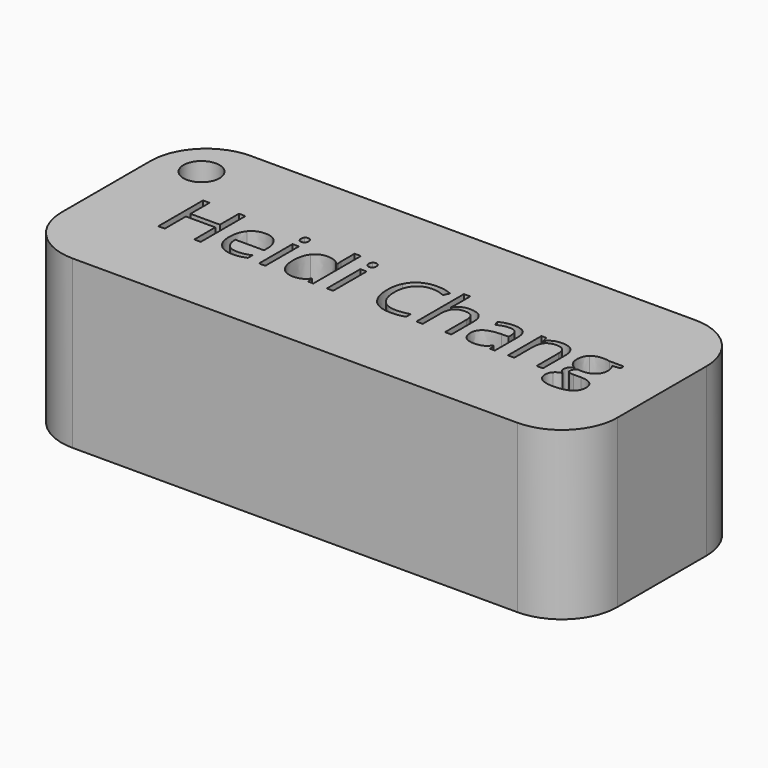
from build123d import *

# Parameters (mm, degrees)
F0_W     = 1.1420084165
F0_H     = 7.5363753885
F0_R     = 3.2310407431
F1_DEPTH = 30


with BuildPart() as f1:
    # F0 (on Top) → F1 (new body)
    with BuildSketch(Plane.XY):
        with BuildLine():
            Line((90, 41.9395349271), (10, 41.9395349271))
            ThreePointArc((10, 41.9395349271), (2.9289321881, 39.0106027389), (0, 31.9395349271))
            Line((0, 31.9395349271), (0, 11.9395349271))
            ThreePointArc((0, 11.9395349271), (2.9289321881, 4.8684671152), (10, 1.9395349271))
            Line((10, 1.9395349271), (90, 1.9395349271))
            ThreePointArc((90, 1.9395349271), (97.0710678119, 4.8684671152), (100, 11.9395349271))
            Line((100, 11.9395349271), (100, 31.9395349271))
            ThreePointArc((100, 31.9395349271), (97.0710678119, 39.0106027389), (90, 41.9395349271))
        make_face()
        with BuildLine():
            add(Edge.make_bspline(
                [(27.9621376159, 17.0902174011), (27.4230392305, 16.9757965193), (26.6594998845, 16.9757965193)],
                knots=[0, 0, 0, 1, 1, 1], degree=2))
            add(Edge.make_bspline(
                [(26.6594998845, 16.9757965193), (24.9893950904, 16.9757965193), (24.022318599, 17.9945824477)],
                knots=[0, 0, 0, 1, 1, 1], degree=2))
            add(Edge.make_bspline(
                [(24.022318599, 17.9945824477), (23.0552421075, 19.0133683762), (23.0552421075, 20.8198980678)],
                knots=[0, 0, 0, 1, 1, 1], degree=2))
            add(Edge.make_bspline(
                [(23.0552421075, 20.8198980678), (23.0552421075, 22.6440309721), (23.9530059494, 23.7167267391)],
                knots=[0, 0, 0, 1, 1, 1], degree=2))
            add(Edge.make_bspline(
                [(23.9530059494, 23.7167267391), (24.8507697913, 24.789422506), (26.3646460737, 24.789422506)],
                knots=[0, 0, 0, 1, 1, 1], degree=2))
            add(Edge.make_bspline(
                [(26.3646460737, 24.789422506), (27.7795042854, 24.789422506), (28.6046548753, 23.8575524397)],
                knots=[0, 0, 0, 1, 1, 1], degree=2))
            add(Edge.make_bspline(
                [(28.6046548753, 23.8575524397), (29.4298054653, 22.9256823735), (29.4298054653, 21.3986036816)],
                knots=[0, 0, 0, 1, 1, 1], degree=2))
            Line((29.4298054653, 21.3986036816), (29.4298054653, 20.6768719656))
            Line((29.4298054653, 20.6768719656), (24.2390581539, 20.6768719656))
            add(Edge.make_bspline(
                [(24.2390581539, 20.6768719656), (24.2742645791, 19.3500298169), (24.9101806338, 18.6624043252)],
                knots=[0, 0, 0, 1, 1, 1], degree=2))
            add(Edge.make_bspline(
                [(24.9101806338, 18.6624043252), (25.5460966885, 17.9747788336), (26.7013075144, 17.9747788336)],
                knots=[0, 0, 0, 1, 1, 1], degree=2))
            add(Edge.make_bspline(
                [(26.7013075144, 17.9747788336), (27.9181295845, 17.9747788336), (29.106346434, 18.483071597)],
                knots=[0, 0, 0, 1, 1, 1], degree=2))
            Line((29.106346434, 18.483071597), (29.106346434, 17.4642856686))
            add(Edge.make_bspline(
                [(29.106346434, 17.4642856686), (28.5012360014, 17.2046382829), (27.9621376159, 17.0902174011)],
                knots=[0, 0, 0, 1, 1, 1], degree=2))
        make_face(mode=Mode.SUBTRACT)
        with Locations((31.9481650659, 20.8826095127)):
            Rectangle(F0_W, F0_H, mode=Mode.SUBTRACT)
        with Locations((44.1405901835, 20.8826095127)):
            Rectangle(F0_W, F0_H, mode=Mode.SUBTRACT)
        with BuildLine():
            Line((73.8009031907, 17.1144218184), (72.9537485849, 17.1144218184))
            Line((72.9537485849, 17.1144218184), (72.7271072229, 18.1882177862))
            Line((72.7271072229, 18.1882177862), (72.6720971836, 18.1882177862))
            add(Edge.make_bspline(
                [(72.6720971836, 18.1882177862), (72.1087943808, 17.4796884796), (71.5487921804, 17.2277424994)],
                knots=[0, 0, 0, 1, 1, 1], degree=2))
            add(Edge.make_bspline(
                [(71.5487921804, 17.2277424994), (70.98878998, 16.9757965193), (70.148236579, 16.9757965193)],
                knots=[0, 0, 0, 1, 1, 1], degree=2))
            add(Edge.make_bspline(
                [(70.148236579, 16.9757965193), (69.0282321782, 16.9757965193), (68.3923161235, 17.5545021331)],
                knots=[0, 0, 0, 1, 1, 1], degree=2))
            add(Edge.make_bspline(
                [(68.3923161235, 17.5545021331), (67.7564000688, 18.1332077468), (67.7564000688, 19.1982021083)],
                knots=[0, 0, 0, 1, 1, 1], degree=2))
            add(Edge.make_bspline(
                [(67.7564000688, 19.1982021083), (67.7564000688, 21.4800185398), (71.4068662789, 21.5900386185)],
                knots=[0, 0, 0, 1, 1, 1], degree=2))
            Line((71.4068662789, 21.5900386185), (72.685299593, 21.6318462484))
            Line((72.685299593, 21.6318462484), (72.685299593, 22.1005317835))
            add(Edge.make_bspline(
                [(72.685299593, 22.1005317835), (72.685299593, 22.9872936175), (72.3046301208, 23.4097707196)],
                knots=[0, 0, 0, 1, 1, 1], degree=2))
            add(Edge.make_bspline(
                [(72.3046301208, 23.4097707196), (71.9239606486, 23.8322478217), (71.0834072476, 23.8322478217)],
                knots=[0, 0, 0, 1, 1, 1], degree=2))
            add(Edge.make_bspline(
                [(71.0834072476, 23.8322478217), (70.1416353743, 23.8322478217), (68.9534185247, 23.2557426094)],
                knots=[0, 0, 0, 1, 1, 1], degree=2))
            Line((68.9534185247, 23.2557426094), (68.601354273, 24.129302034))
            add(Edge.make_bspline(
                [(68.601354273, 24.129302034), (69.158055871, 24.4307570496), (69.8214769454, 24.6023883723)],
                knots=[0, 0, 0, 1, 1, 1], degree=2))
            add(Edge.make_bspline(
                [(69.8214769454, 24.6023883723), (70.4848980197, 24.774019695), (71.153820098, 24.774019695)],
                knots=[0, 0, 0, 1, 1, 1], degree=2))
            add(Edge.make_bspline(
                [(71.153820098, 24.774019695), (72.5004658608, 24.774019695), (73.1506845257, 24.1766106679)],
                knots=[0, 0, 0, 1, 1, 1], degree=2))
            add(Edge.make_bspline(
                [(73.1506845257, 24.1766106679), (73.8009031907, 23.5792016407), (73.8009031907, 22.2589606968)],
                knots=[0, 0, 0, 1, 1, 1], degree=2))
            Line((73.8009031907, 22.2589606968), (73.8009031907, 17.1144218184))
        make_face(mode=Mode.SUBTRACT)
        with BuildLine():
            Line((88.3565595979, 24.6507972069), (90.9618350607, 24.6507972069))
            Line((90.9618350607, 24.6507972069), (90.9618350607, 23.9290654909))
            Line((90.9618350607, 23.9290654909), (89.5667804633, 23.7640353729))
            add(Edge.make_bspline(
                [(89.5667804633, 23.7640353729), (89.7582154001, 23.5241916014), (89.9100431087, 23.1347205229)],
                knots=[0, 0, 0, 1, 1, 1], degree=2))
            add(Edge.make_bspline(
                [(89.9100431087, 23.1347205229), (90.0618708172, 22.7452494444), (90.0618708172, 22.2589606968)],
                knots=[0, 0, 0, 1, 1, 1], degree=2))
            add(Edge.make_bspline(
                [(90.0618708172, 22.2589606968), (90.0618708172, 21.1499583038), (89.304932676, 20.4898378318)],
                knots=[0, 0, 0, 1, 1, 1], degree=2))
            add(Edge.make_bspline(
                [(89.304932676, 20.4898378318), (88.5479945348, 19.8297173598), (87.2277535909, 19.8297173598)],
                knots=[0, 0, 0, 1, 1, 1], degree=2))
            add(Edge.make_bspline(
                [(87.2277535909, 19.8297173598), (86.8910921501, 19.8297173598), (86.5962383393, 19.8847273992)],
                knots=[0, 0, 0, 1, 1, 1], degree=2))
            add(Edge.make_bspline(
                [(86.5962383393, 19.8847273992), (85.8679054186, 19.4996571238), (85.8679054186, 18.9165507069)],
                knots=[0, 0, 0, 1, 1, 1], degree=2))
            add(Edge.make_bspline(
                [(85.8679054186, 18.9165507069), (85.8679054186, 18.6062940851), (86.1220518003, 18.4588671797)],
                knots=[0, 0, 0, 1, 1, 1], degree=2))
            add(Edge.make_bspline(
                [(86.1220518003, 18.4588671797), (86.376198182, 18.3114402743), (86.9945110241, 18.3114402743)],
                knots=[0, 0, 0, 1, 1, 1], degree=2))
            Line((86.9945110241, 18.3114402743), (88.3279543775, 18.3114402743))
            add(Edge.make_bspline(
                [(88.3279543775, 18.3114402743), (89.5535780538, 18.3114402743), (90.2092977227, 17.7954461053)],
                knots=[0, 0, 0, 1, 1, 1], degree=2))
            add(Edge.make_bspline(
                [(90.2092977227, 17.7954461053), (90.8650173915, 17.2794519364), (90.8650173915, 16.2958724331)],
                knots=[0, 0, 0, 1, 1, 1], degree=2))
            add(Edge.make_bspline(
                [(90.8650173915, 16.2958724331), (90.8650173915, 15.0438439379), (89.8616342741, 14.3870240683)],
                knots=[0, 0, 0, 1, 1, 1], degree=2))
            add(Edge.make_bspline(
                [(89.8616342741, 14.3870240683), (88.8582511567, 13.7302041987), (86.93289978, 13.7302041987)],
                knots=[0, 0, 0, 1, 1, 1], degree=2))
            add(Edge.make_bspline(
                [(86.93289978, 13.7302041987), (85.4542299228, 13.7302041987), (84.6532837501, 14.280304592)],
                knots=[0, 0, 0, 1, 1, 1], degree=2))
            add(Edge.make_bspline(
                [(84.6532837501, 14.280304592), (83.8523375774, 14.8304049853), (83.8523375774, 15.8359885043)],
                knots=[0, 0, 0, 1, 1, 1], degree=2))
            add(Edge.make_bspline(
                [(83.8523375774, 15.8359885043), (83.8523375774, 16.5225137952), (84.2924178921, 17.0253055547)],
                knots=[0, 0, 0, 1, 1, 1], degree=2))
            add(Edge.make_bspline(
                [(84.2924178921, 17.0253055547), (84.7324982067, 17.5280973142), (85.5290435763, 17.7063298416)],
                knots=[0, 0, 0, 1, 1, 1], degree=2))
            add(Edge.make_bspline(
                [(85.5290435763, 17.7063298416), (85.2407909702, 17.8361535344), (85.0449552302, 18.1112037311)],
                knots=[0, 0, 0, 1, 1, 1], degree=2))
            add(Edge.make_bspline(
                [(85.0449552302, 18.1112037311), (84.8491194901, 18.3862539278), (84.8491194901, 18.7515205889)],
                knots=[0, 0, 0, 1, 1, 1], degree=2))
            add(Edge.make_bspline(
                [(84.8491194901, 18.7515205889), (84.8491194901, 19.1629956831), (85.0691596475, 19.473252305)],
                knots=[0, 0, 0, 1, 1, 1], degree=2))
            add(Edge.make_bspline(
                [(85.0691596475, 19.473252305), (85.2891998048, 19.7835089268), (85.7644865446, 20.0717615329)],
                knots=[0, 0, 0, 1, 1, 1], degree=2))
            add(Edge.make_bspline(
                [(85.7644865446, 20.0717615329), (85.1791797261, 20.3116053044), (84.8117126634, 20.8892107174)],
                knots=[0, 0, 0, 1, 1, 1], degree=2))
            add(Edge.make_bspline(
                [(84.8117126634, 20.8892107174), (84.4442456006, 21.4668161304), (84.4442456006, 22.2105518621)],
                knots=[0, 0, 0, 1, 1, 1], degree=2))
            add(Edge.make_bspline(
                [(84.4442456006, 22.2105518621), (84.4442456006, 23.4471775463), (85.1868811316, 24.1183000262)],
                knots=[0, 0, 0, 1, 1, 1], degree=2))
            add(Edge.make_bspline(
                [(85.1868811316, 24.1183000262), (85.9295166626, 24.789422506), (87.2893648349, 24.789422506)],
                knots=[0, 0, 0, 1, 1, 1], degree=2))
            add(Edge.make_bspline(
                [(87.2893648349, 24.789422506), (87.8812728581, 24.789422506), (88.3565595979, 24.6507972069)],
                knots=[0, 0, 0, 1, 1, 1], degree=2))
        make_face(mode=Mode.SUBTRACT)
        with BuildLine():
            Line((82.4506817752, 17.1144218184), (81.3086733587, 17.1144218184))
            Line((81.3086733587, 17.1144218184), (81.3086733587, 21.9905117048))
            add(Edge.make_bspline(
                [(81.3086733587, 21.9905117048), (81.3086733587, 22.9102795624), (80.889496859, 23.3646624873)],
                knots=[0, 0, 0, 1, 1, 1], degree=2))
            add(Edge.make_bspline(
                [(80.889496859, 23.3646624873), (80.4703203593, 23.8190454122), (79.574756919, 23.8190454122)],
                knots=[0, 0, 0, 1, 1, 1], degree=2))
            add(Edge.make_bspline(
                [(79.574756919, 23.8190454122), (78.3931412741, 23.8190454122), (77.8430408808, 23.1798287552)],
                knots=[0, 0, 0, 1, 1, 1], degree=2))
            add(Edge.make_bspline(
                [(77.8430408808, 23.1798287552), (77.2929404875, 22.5406120981), (77.2929404875, 21.0685434456)],
                knots=[0, 0, 0, 1, 1, 1], degree=2))
            Line((77.2929404875, 21.0685434456), (77.2929404875, 17.1144218184))
            Line((77.2929404875, 17.1144218184), (76.1509320709, 17.1144218184))
            Line((76.1509320709, 17.1144218184), (76.1509320709, 24.6507972069))
            Line((76.1509320709, 24.6507972069), (77.0795015349, 24.6507972069))
            Line((77.0795015349, 24.6507972069), (77.264335267, 23.618808869))
            Line((77.264335267, 23.618808869), (77.3193453063, 23.618808869))
            add(Edge.make_bspline(
                [(77.3193453063, 23.618808869), (77.6714095581, 24.1755104671), (78.3040250104, 24.4824664866)],
                knots=[0, 0, 0, 1, 1, 1], degree=2))
            add(Edge.make_bspline(
                [(78.3040250104, 24.4824664866), (78.9366404627, 24.789422506), (79.7133822181, 24.789422506)],
                knots=[0, 0, 0, 1, 1, 1], degree=2))
            add(Edge.make_bspline(
                [(79.7133822181, 24.789422506), (81.0754307919, 24.789422506), (81.7630562836, 24.1326026364)],
                knots=[0, 0, 0, 1, 1, 1], degree=2))
            add(Edge.make_bspline(
                [(81.7630562836, 24.1326026364), (82.4506817752, 23.4757827668), (82.4506817752, 22.0301189331)],
                knots=[0, 0, 0, 1, 1, 1], degree=2))
            Line((82.4506817752, 22.0301189331), (82.4506817752, 17.1144218184))
        make_face(mode=Mode.SUBTRACT)
        Polygon((20.8900469594, 27.1680566068), (20.8900469594, 17.1144218184), (19.721633724, 17.1144218184), (19.721633724, 21.845285201), (14.4252671371, 21.845285201), (14.4252671371, 17.1144218184), (13.2568539017, 17.1144218184), (13.2568539017, 27.1680566068), (14.4252671371, 27.1680566068), (14.4252671371, 22.8904759483), (19.721633724, 22.8904759483), (19.721633724, 27.1680566068), align=None, mode=Mode.SUBTRACT)
        with BuildLine():
            add(Edge.make_bspline(
                [(31.4728783261, 26.1184650563), (31.2803431885, 26.3076995916), (31.2803431885, 26.6927698669)],
                knots=[0, 0, 0, 1, 1, 1], degree=2))
            add(Edge.make_bspline(
                [(31.2803431885, 26.6927698669), (31.2803431885, 27.084441347), (31.4728783261, 27.2670746776)],
                knots=[0, 0, 0, 1, 1, 1], degree=2))
            add(Edge.make_bspline(
                [(31.4728783261, 27.2670746776), (31.6654134638, 27.4497080081), (31.9558664715, 27.4497080081)],
                knots=[0, 0, 0, 1, 1, 1], degree=2))
            add(Edge.make_bspline(
                [(31.9558664715, 27.4497080081), (32.2309166681, 27.4497080081), (32.4300530105, 27.2637740752)],
                knots=[0, 0, 0, 1, 1, 1], degree=2))
            add(Edge.make_bspline(
                [(32.4300530105, 27.2637740752), (32.6291893529, 27.0778401422), (32.6291893529, 26.6927698669)],
                knots=[0, 0, 0, 1, 1, 1], degree=2))
            add(Edge.make_bspline(
                [(32.6291893529, 26.6927698669), (32.6291893529, 26.3076995916), (32.4300530105, 26.1184650563)],
                knots=[0, 0, 0, 1, 1, 1], degree=2))
            add(Edge.make_bspline(
                [(32.4300530105, 26.1184650563), (32.2309166681, 25.929230521), (31.9558664715, 25.929230521)],
                knots=[0, 0, 0, 1, 1, 1], degree=2))
            add(Edge.make_bspline(
                [(31.9558664715, 25.929230521), (31.6654134638, 25.929230521), (31.4728783261, 26.1184650563)],
                knots=[0, 0, 0, 1, 1, 1], degree=2))
        make_face(mode=Mode.SUBTRACT)
        with BuildLine():
            Line((40.2205747807, 17.1144218184), (40.0687470722, 18.1244061405))
            Line((40.0687470722, 18.1244061405), (40.0071358281, 18.1244061405))
            add(Edge.make_bspline(
                [(40.0071358281, 18.1244061405), (39.2171916633, 16.9757965193), (37.6417041368, 16.9757965193)],
                knots=[0, 0, 0, 1, 1, 1], degree=2))
            add(Edge.make_bspline(
                [(37.6417041368, 16.9757965193), (36.1630342796, 16.9757965193), (35.341184292, 17.9868810422)],
                knots=[0, 0, 0, 1, 1, 1], degree=2))
            add(Edge.make_bspline(
                [(35.341184292, 17.9868810422), (34.5193343043, 18.9979655651), (34.5193343043, 20.8617056977)],
                knots=[0, 0, 0, 1, 1, 1], degree=2))
            add(Edge.make_bspline(
                [(34.5193343043, 20.8617056977), (34.5193343043, 22.7254458303), (35.3444848943, 23.7574341682)],
                knots=[0, 0, 0, 1, 1, 1], degree=2))
            add(Edge.make_bspline(
                [(35.3444848943, 23.7574341682), (36.1696354843, 24.789422506), (37.6417041368, 24.789422506)],
                knots=[0, 0, 0, 1, 1, 1], degree=2))
            add(Edge.make_bspline(
                [(37.6417041368, 24.789422506), (39.1753840334, 24.789422506), (39.9939334187, 23.6738189084)],
                knots=[0, 0, 0, 1, 1, 1], degree=2))
            Line((39.9939334187, 23.6738189084), (40.0841498832, 23.6738189084))
            Line((40.0841498832, 23.6738189084), (40.0357410486, 24.217318097))
            Line((40.0357410486, 24.217318097), (40.0071358281, 24.7476148761))
            Line((40.0071358281, 24.7476148761), (40.0071358281, 27.8149746693))
            Line((40.0071358281, 27.8149746693), (41.1491442446, 27.8149746693))
            Line((41.1491442446, 27.8149746693), (41.1491442446, 17.1144218184))
            Line((41.1491442446, 17.1144218184), (40.2205747807, 17.1144218184))
        make_face(mode=Mode.SUBTRACT)
        with BuildLine():
            add(Edge.make_bspline(
                [(43.6653034437, 26.1184650563), (43.472768306, 26.3076995916), (43.472768306, 26.6927698669)],
                knots=[0, 0, 0, 1, 1, 1], degree=2))
            add(Edge.make_bspline(
                [(43.472768306, 26.6927698669), (43.472768306, 27.084441347), (43.6653034437, 27.2670746776)],
                knots=[0, 0, 0, 1, 1, 1], degree=2))
            add(Edge.make_bspline(
                [(43.6653034437, 27.2670746776), (43.8578385814, 27.4497080081), (44.148291589, 27.4497080081)],
                knots=[0, 0, 0, 1, 1, 1], degree=2))
            add(Edge.make_bspline(
                [(44.148291589, 27.4497080081), (44.4233417857, 27.4497080081), (44.6224781281, 27.2637740752)],
                knots=[0, 0, 0, 1, 1, 1], degree=2))
            add(Edge.make_bspline(
                [(44.6224781281, 27.2637740752), (44.8216144705, 27.0778401422), (44.8216144705, 26.6927698669)],
                knots=[0, 0, 0, 1, 1, 1], degree=2))
            add(Edge.make_bspline(
                [(44.8216144705, 26.6927698669), (44.8216144705, 26.3076995916), (44.6224781281, 26.1184650563)],
                knots=[0, 0, 0, 1, 1, 1], degree=2))
            add(Edge.make_bspline(
                [(44.6224781281, 26.1184650563), (44.4233417857, 25.929230521), (44.148291589, 25.929230521)],
                knots=[0, 0, 0, 1, 1, 1], degree=2))
            add(Edge.make_bspline(
                [(44.148291589, 25.929230521), (43.8578385814, 25.929230521), (43.6653034437, 26.1184650563)],
                knots=[0, 0, 0, 1, 1, 1], degree=2))
        make_face(mode=Mode.SUBTRACT)
        with Locations((7.624998223, 33.8764637709)):
            Circle(F0_R, mode=Mode.SUBTRACT)
        with BuildLine():
            add(Edge.make_bspline(
                [(57.5509375719, 25.7311943794), (56.4089291554, 26.2658919617), (55.2669207389, 26.2658919617)],
                knots=[0, 0, 0, 1, 1, 1], degree=2))
            add(Edge.make_bspline(
                [(55.2669207389, 26.2658919617), (53.6100183542, 26.2658919617), (52.6506432682, 25.1623905727)],
                knots=[0, 0, 0, 1, 1, 1], degree=2))
            add(Edge.make_bspline(
                [(52.6506432682, 25.1623905727), (51.6912681823, 24.0588891837), (51.6912681823, 22.1401390118)],
                knots=[0, 0, 0, 1, 1, 1], degree=2))
            add(Edge.make_bspline(
                [(51.6912681823, 22.1401390118), (51.6912681823, 20.1685792021), (52.6165370438, 19.091482632)],
                knots=[0, 0, 0, 1, 1, 1], degree=2))
            add(Edge.make_bspline(
                [(52.6165370438, 19.091482632), (53.5418059054, 18.0143860619), (55.2537183294, 18.0143860619)],
                knots=[0, 0, 0, 1, 1, 1], degree=2))
            add(Edge.make_bspline(
                [(55.2537183294, 18.0143860619), (56.3055102814, 18.0143860619), (57.6543564459, 18.3928551325)],
                knots=[0, 0, 0, 1, 1, 1], degree=2))
            Line((57.6543564459, 18.3928551325), (57.6543564459, 17.3696684009))
            add(Edge.make_bspline(
                [(57.6543564459, 17.3696684009), (56.6091656986, 16.9757965193), (55.075485802, 16.9757965193)],
                knots=[0, 0, 0, 1, 1, 1], degree=2))
            add(Edge.make_bspline(
                [(55.075485802, 16.9757965193), (52.8552806145, 16.9757965193), (51.6483603516, 18.3246426837)],
                knots=[0, 0, 0, 1, 1, 1], degree=2))
            add(Edge.make_bspline(
                [(51.6483603516, 18.3246426837), (50.4414400886, 19.6734888481), (50.4414400886, 22.1555418228)],
                knots=[0, 0, 0, 1, 1, 1], degree=2))
            add(Edge.make_bspline(
                [(50.4414400886, 22.1555418228), (50.4414400886, 23.7090253335), (51.022346104, 24.877438569)],
                knots=[0, 0, 0, 1, 1, 1], degree=2))
            add(Edge.make_bspline(
                [(51.022346104, 24.877438569), (51.6032521193, 26.0458518044), (52.7001523036, 26.6784672567)],
                knots=[0, 0, 0, 1, 1, 1], degree=2))
            add(Edge.make_bspline(
                [(52.7001523036, 26.6784672567), (53.7970524879, 27.311082709), (55.2823235499, 27.311082709)],
                knots=[0, 0, 0, 1, 1, 1], degree=2))
            add(Edge.make_bspline(
                [(55.2823235499, 27.311082709), (56.8622118795, 27.311082709), (58.0460279259, 26.7345774968)],
                knots=[0, 0, 0, 1, 1, 1], degree=2))
            Line((58.0460279259, 26.7345774968), (57.5509375719, 25.7311943794))
        make_face(mode=Mode.SUBTRACT)
        with BuildLine():
            Line((65.976275196, 17.1144218184), (64.8342667795, 17.1144218184))
            Line((64.8342667795, 17.1144218184), (64.8342667795, 21.9905117048))
            add(Edge.make_bspline(
                [(64.8342667795, 21.9905117048), (64.8342667795, 22.9102795624), (64.4150902798, 23.3646624873)],
                knots=[0, 0, 0, 1, 1, 1], degree=2))
            add(Edge.make_bspline(
                [(64.4150902798, 23.3646624873), (63.9959137801, 23.8190454122), (63.1003503398, 23.8190454122)],
                knots=[0, 0, 0, 1, 1, 1], degree=2))
            add(Edge.make_bspline(
                [(63.1003503398, 23.8190454122), (61.9121334902, 23.8190454122), (61.3653336992, 23.1721273497)],
                knots=[0, 0, 0, 1, 1, 1], degree=2))
            add(Edge.make_bspline(
                [(61.3653336992, 23.1721273497), (60.8185339083, 22.5252092871), (60.8185339083, 21.0553410362)],
                knots=[0, 0, 0, 1, 1, 1], degree=2))
            Line((60.8185339083, 21.0553410362), (60.8185339083, 17.1144218184))
            Line((60.8185339083, 17.1144218184), (59.6765254917, 17.1144218184))
            Line((59.6765254917, 17.1144218184), (59.6765254917, 27.8149746693))
            Line((59.6765254917, 27.8149746693), (60.8185339083, 27.8149746693))
            Line((60.8185339083, 27.8149746693), (60.8185339083, 24.5759835534))
            add(Edge.make_bspline(
                [(60.8185339083, 24.5759835534), (60.8185339083, 23.9906767349), (60.7635238689, 23.6056064596)],
                knots=[0, 0, 0, 1, 1, 1], degree=2))
            Line((60.7635238689, 23.6056064596), (60.8317363177, 23.6056064596))
            add(Edge.make_bspline(
                [(60.8317363177, 23.6056064596), (61.1683977584, 24.1491056482), (61.7911114037, 24.4615626716)],
                knots=[0, 0, 0, 1, 1, 1], degree=2))
            add(Edge.make_bspline(
                [(61.7911114037, 24.4615626716), (62.4138250489, 24.774019695), (63.2103704184, 24.774019695)],
                knots=[0, 0, 0, 1, 1, 1], degree=2))
            add(Edge.make_bspline(
                [(63.2103704184, 24.774019695), (64.5922226064, 24.774019695), (65.2842489012, 24.1171998254)],
                knots=[0, 0, 0, 1, 1, 1], degree=2))
            add(Edge.make_bspline(
                [(65.2842489012, 24.1171998254), (65.976275196, 23.4603799558), (65.976275196, 22.0301189331)],
                knots=[0, 0, 0, 1, 1, 1], degree=2))
            Line((65.976275196, 22.0301189331), (65.976275196, 17.1144218184))
        make_face(mode=Mode.SUBTRACT)
    extrude(amount=F1_DEPTH)


solid = f1.part
